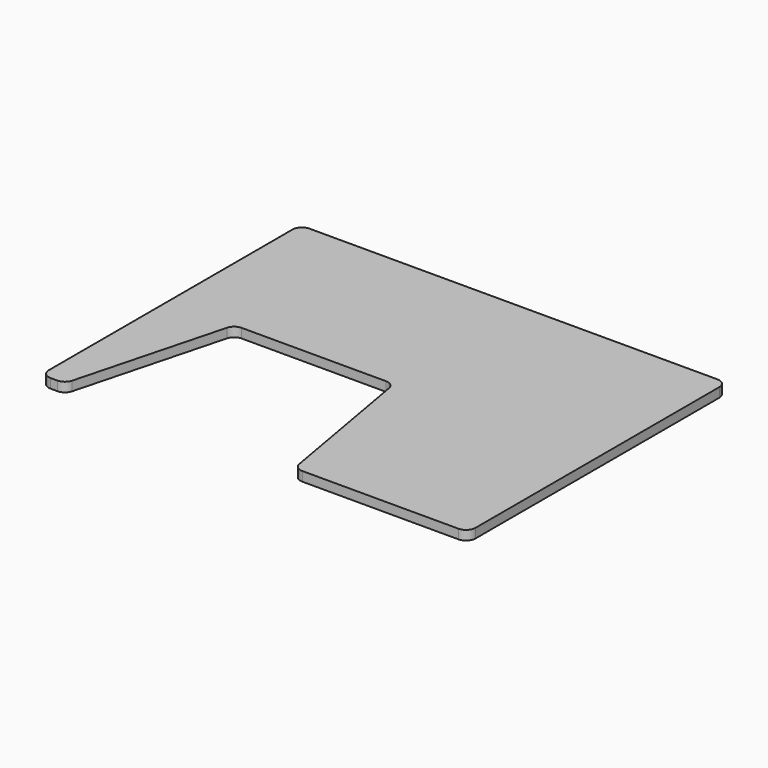
from build123d import *

# Parameters (mm, degrees)
F0_W     = 910
F0_H     = 690
F1_DEPTH = 20
F2_W     = 340
F2_H     = 340
F3_DEPTH = 25
F4_R     = 20


with BuildPart() as f1:
    # F0 (on Top) → F1 (new body)
    with BuildSketch(Plane.XY):
        Rectangle(F0_W, F0_H)
    extrude(amount=F1_DEPTH)

    # F2 (on face) → F3 (cut)
    with BuildSketch(Plane.XY.offset(20)):
        with Locations((-145, -175)):
            Rectangle(F2_W, F2_H)
        Polygon((-405, -345), (-315, -345), (-315, -5), align=None)
        Polygon((25, -5), (25, -345), (85, -345), align=None)
    extrude(amount=-F3_DEPTH, mode=Mode.SUBTRACT)

    # F4
    f4_edges = [f1.edges().sort_by_distance(p)[0] for p in [
        (-315, -5, 10),
        (25, -5, 10),
        (455, -345, 10),
        (455, 345, 10),
        (-455, 345, 10),
        (-455, -345, 10),
        (-405, -345, 10),
        (85, -345, 10),
    ]]
    fillet(f4_edges, radius=F4_R)


solid = f1.part
